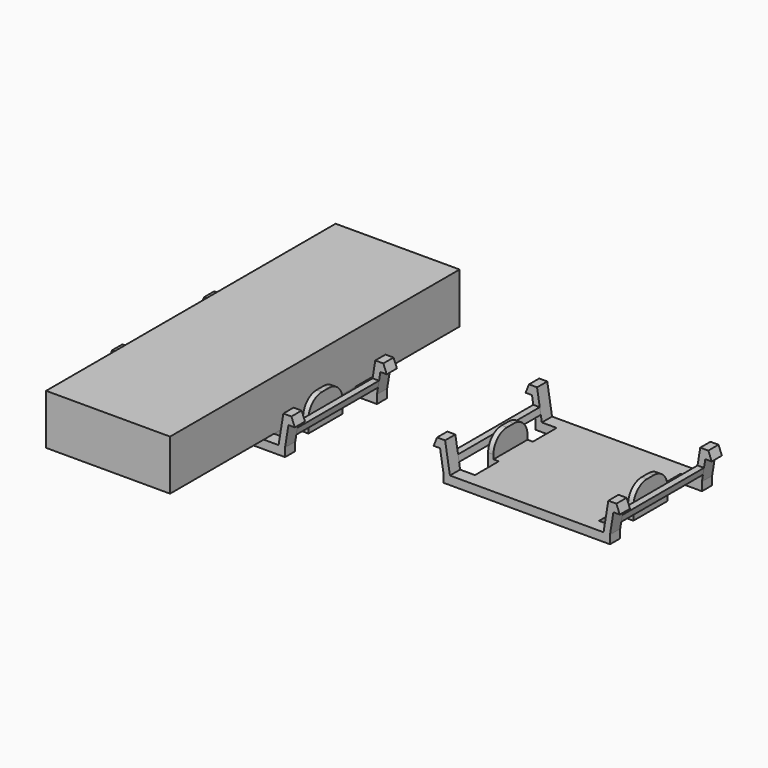
from build123d import *

# Parameters (mm, degrees)
F0_W             = 37
F0_H             = 108
F1_DEPTH         = 15
F2_W             = 6.35
F2_H             = 3.81
F2_W_2           = 3.175
F2_H_2           = 12.7
F3_DEPTH         = 2.54
F4_W             = 1.5875
F4_H             = 12.7
F5_DEPTH         = 6.35
F6_R             = 5.08
F8_DEPTH         = 3.81
F8_COPIES2_COUNT = 2
F10_DEPTH        = 15.24


# Not quite as in the source:
# - a pattern or mirror of a feature is missing from the dataset's text; its kind, count and spacing are read off the source's solid


with BuildPart() as f1:
    # F0 (on Top) → F1 (new body)
    with BuildSketch(Plane.XY):
        Rectangle(F0_W, F0_H)
    extrude(amount=F1_DEPTH)


with BuildPart() as f3:
    # F2 (on Top) → F3 (new body)
    with BuildSketch(Plane.XY):
        Polygon((-18.5, -19.05), (18.5, -19.05), (18.5, -15.24), (18.5, -6.35), (15.325, -6.35), (15.325, 6.35), (18.5, 6.35), (18.5, 15.24), (18.5, 19.05), (-18.5, 19.05), (-18.5, 15.24), (-18.5, 6.35), (-15.325, 6.35), (-15.325, -6.35), (-18.5, -6.35), (-18.5, -15.24), align=None)
        with Locations((21.675, -17.145)):
            Rectangle(F2_W, F2_H)
        with Locations((-21.675, -17.145)):
            Rectangle(F2_W, F2_H)
        with Locations((16.9125, 0)):
            Rectangle(F2_W_2, F2_H_2)
        with Locations((20.0875, 0)):
            Rectangle(F2_W_2, F2_H_2)
        with Locations((-20.0875, 0)):
            Rectangle(F2_W_2, F2_H_2)
        with Locations((-16.9125, 0)):
            Rectangle(F2_W_2, F2_H_2)
        with Locations((21.675, 17.145)):
            Rectangle(F2_W, F2_H)
        with Locations((-21.675, 17.145)):
            Rectangle(F2_W, F2_H)
    extrude(amount=-F3_DEPTH)

    # F4 (on face) → F5 (join)
    with BuildSketch(Plane.XY):
        with Locations((-20.88125, 0)):
            Rectangle(F4_W, F4_H)
        with Locations((20.88125, 0)):
            Rectangle(F4_W, F4_H)
    extrude(amount=F5_DEPTH)

    # F6
    f6_edges = [f3.edges().sort_by_distance(p)[0] for p in [
        (-20.88125, -6.35, 6.35),
        (-20.88125, 6.35, 6.35),
        (20.88125, -6.35, 6.35),
        (20.88125, 6.35, 6.35),
    ]]
    fillet(f6_edges, radius=F6_R)

    # F7 (on face) → F8 (join)
    with BuildSketch(Plane.XZ.offset(19.05)):
        Polygon((-25.866, 6.223), (-24.85, 0), (-22.9197775532, 0), (-24.3504714307, 8.763), (-26.755, 8.763), (-27.771, 6.223), align=None)
    f8 = extrude(amount=-F8_DEPTH)

    # F8_copies: F8 across plane
    add(f8.mirror(Plane.ZX))

    # F8_copies1: F8 across plane
    add(f8.mirror(Plane(origin=(0, 0, 0), x_dir=(0, 0, 1), z_dir=(1, 0, 0))))

    # F8_copies2: F8 ×2 about axis
    f8_copies2_axis = Axis((0, 0, 0), (0, 0, 1))
    for i in range(1, F8_COPIES2_COUNT):
        add(f8.rotate(f8_copies2_axis, i * 360 / F8_COPIES2_COUNT))

    # F9 (on Front) → F10 (join, symmetric)
    with BuildSketch(Plane.XZ):
        Polygon((-25.4720408163, 3.81), (-25.1610204082, 1.905), (-23.2307979613, 1.905), (-23.5418183695, 3.81), align=None)
        Polygon((23.2307979613, 1.905), (25.1610204082, 1.905), (25.4720408163, 3.81), (23.5418183695, 3.81), align=None)
    extrude(amount=F10_DEPTH, both=True)


with BuildPart() as f11_1:
    # F11: copy of F3
    add(f3.part.moved(Location((86.614, 12.954, 0))))


solid = Compound([f1.part, f3.part, f11_1.part])
